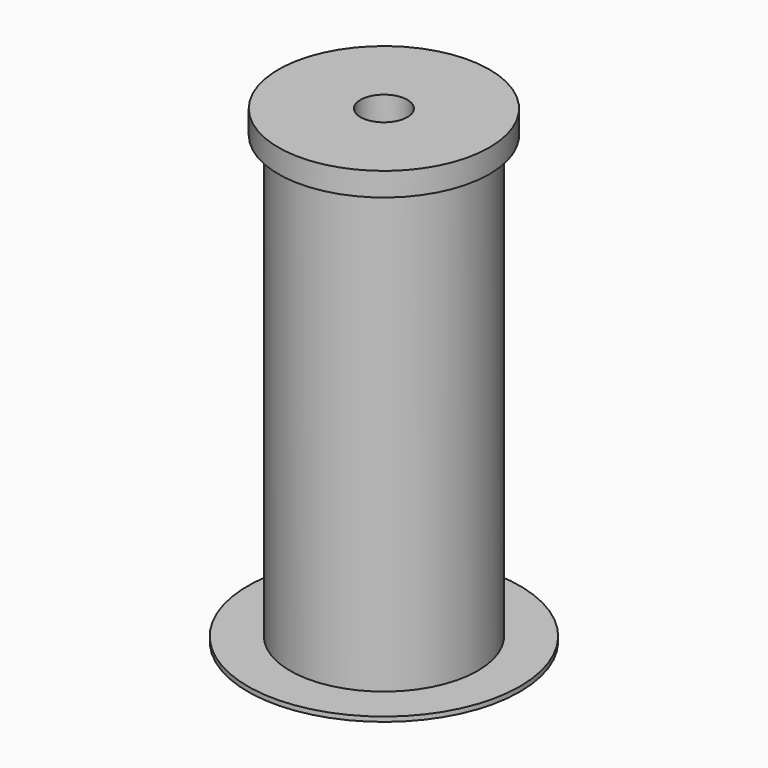
from build123d import *

# Parameters (mm, degrees)
F0_R     = 20
F1_DEPTH = 100
F0_R_2   = 29
F2_DEPTH = 1
F4_R     = 22.5
F4_R_2   = 20
F4_R_3   = 5
F5_DEPTH = 5
F6_DEPTH = 10


# Not quite as in the source:
# - the program builds the solid bodies; features that only make, move or delete a surface that nothing else refers to are left out


with BuildPart() as f1:
    # F0 (on Top) → F1 (new body)
    with BuildSketch(Plane.XY):
        Circle(F0_R)
    extrude(amount=F1_DEPTH)

    # F4 (on face) → F5 (join)
    with BuildSketch(Plane.XY.offset(100)):
        Circle(F4_R)
        Circle(F4_R_2, mode=Mode.SUBTRACT)
        Circle(F4_R_2)
        Circle(F4_R_3, mode=Mode.SUBTRACT)
    extrude(amount=-F5_DEPTH)

    # F4 (on face) → F6 (cut)
    with BuildSketch(Plane.XY.offset(100)):
        Circle(F4_R_3)
    extrude(amount=-F6_DEPTH, mode=Mode.SUBTRACT)


with BuildPart() as f2:
    # F0 (on Top) → F2 (new body)
    with BuildSketch(Plane.XY):
        Circle(F0_R_2)
        Circle(F0_R, mode=Mode.SUBTRACT)
    extrude(amount=F2_DEPTH)


solid = Compound([f1.part, f2.part])
